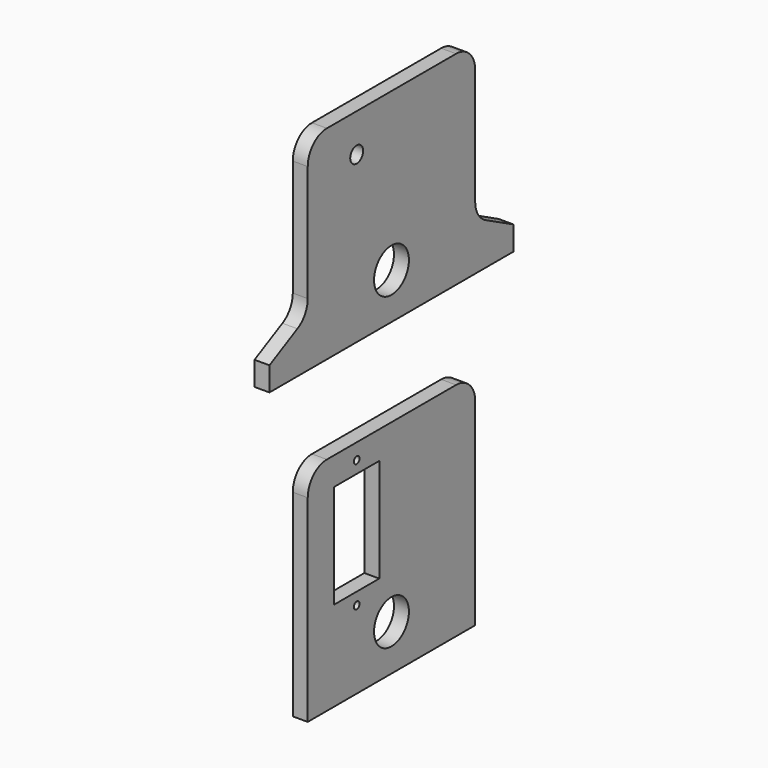
from build123d import *

# Parameters (mm, degrees)
F0_R     = 4.625
F0_R_2   = 1.7145
F1_DEPTH = 3.175
F0_R_3   = 0.75
F0_W     = 12
F0_H     = 5.15
F2_R     = 5.08
F2_2_R   = 5.08


# Not quite as in the source:
# - a feature names something its author has since deleted; it is built from what else it names


with BuildPart() as f1:
    # F0 (on Right) → F1 (new body)
    with BuildSketch(Plane.YZ):
        Polygon((-72.304546833, 31.5911603894), (-72.304546833, 21.2748162448), (-27.854546833, 21.2748162448), (-27.854546833, 31.5911603894), (-27.854546833, 64.4548162448), (-59.604546833, 64.4548162448), (-61.3806888302, 64.4548162448), (-72.304546833, 64.4548162448), align=None)
        with Locations((-50.079546833, 30.9798162448)):
            Circle(F0_R, mode=Mode.SUBTRACT)
        with Locations((-59.3140907028, 56.3515170061)):
            Circle(F0_R_2, mode=Mode.SUBTRACT)
        Polygon((-74.844546833, 21.2748162448), (-72.304546833, 21.2748162448), (-72.304546833, 31.5911603894), (-82.464546833, 26.3548162448), (-82.464546833, 21.2748162448), (-77.384546833, 21.2748162448), align=None)
        Polygon((-27.854546833, 31.5911603894), (-27.854546833, 21.2748162448), (-17.694546833, 21.2748162448), (-17.694546833, 26.3548162448), align=None)
    extrude(amount=F1_DEPTH)

    # F2
    f2_edges = [f1.edges().sort_by_distance(p)[0] for p in [
        (1.5875, -72.304547, 64.454816),
        (1.5875, -72.304547, 31.59116),
        (1.5875, -27.854547, 64.454816),
        (1.5875, -27.854547, 31.59116),
    ]]
    fillet(f2_edges, radius=F2_R)


with BuildPart() as f1b:
    # F0 (on Right) → F1, piece 2 (new body)
    with BuildSketch(Plane.YZ):
        Polygon((-27.854546833, 2.5541710758), (-72.304546833, 2.5541710758), (-72.304546833, -44.4358289242), (-27.854546833, -44.4358289242), (-27.854546833, -41.2608289242), align=None)
        Polygon((-53.3140907028, -9.359128163), (-53.3140907028, -25.359128163), (-53.3140907028, -30.509128163), (-65.3140907028, -30.509128163), (-65.3140907028, -25.359128163), (-65.3140907028, -9.359128163), (-65.3140907028, -3.359128163), (-65.3140907028, 1.790871837), (-53.3140907028, 1.790871837), (-53.3140907028, -3.359128163), align=None, mode=Mode.SUBTRACT)
        with Locations((-50.079546833, -34.7308289242)):
            Circle(F0_R, mode=Mode.SUBTRACT)
        Polygon((-59.3140907028, -3.359128163), (-53.3140907028, -3.359128163), (-53.3140907028, 1.790871837), (-65.3140907028, 1.790871837), (-65.3140907028, -3.359128163), align=None)
        with Locations((-59.3140907028, -0.784128163)):
            Circle(F0_R_3, mode=Mode.SUBTRACT)
        with Locations((-59.3140907028, -27.934128163)):
            Rectangle(F0_W, F0_H)
        with Locations((-59.3140907028, -27.934128163)):
            Circle(F0_R_3, mode=Mode.SUBTRACT)
    extrude(amount=F1_DEPTH)

    # F2#2
    f2_2_edges = [f1b.edges().sort_by_distance(p)[0] for p in [
        (1.5875, -72.304547, 2.554171),
        (1.5875, -27.854547, 2.554171),
    ]]
    fillet(f2_2_edges, radius=F2_2_R)


solid = Compound([f1.part, f1b.part])
